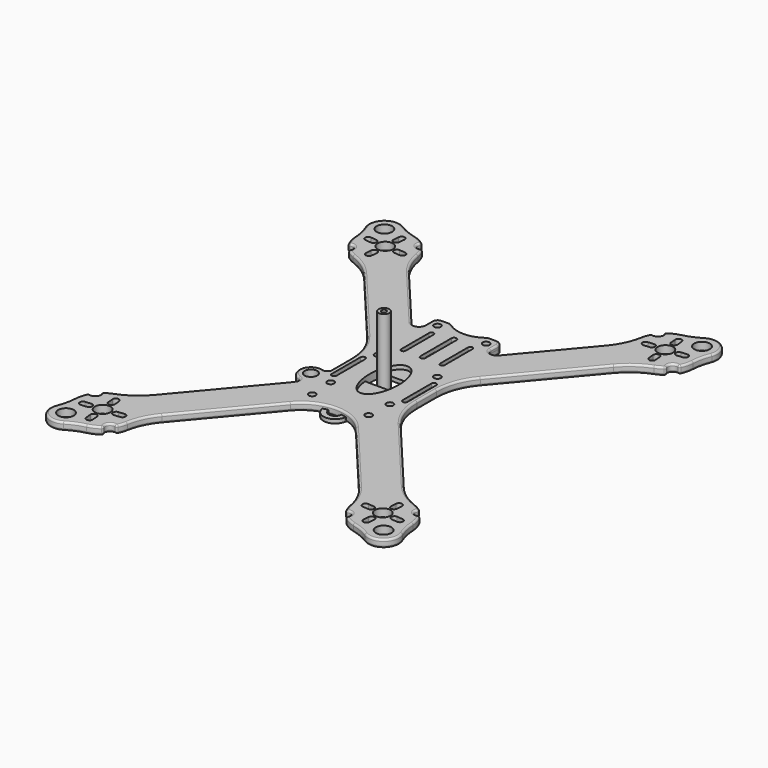
from build123d import *

# Parameters (mm, degrees)
F0_R      = 4
F0_R_2    = 1.75
F0_R_3    = 3.25
F1_DEPTH  = 4
F2_R      = 1
F4_DEPTH  = 25
F6_DEPTH  = 25
F8_DEPTH  = 25
F9_R      = 1.75
F9_R_2    = 3.25
F10_DEPTH = 2
F11_R     = 2.75
F11_R_2   = 1.25
F12_DEPTH = 35
F13_R     = 3
F15_DEPTH = 25


with BuildPart() as f1:
    # F0 (on Top) → F1 (new body)
    with BuildSketch(Plane.XY):
        with BuildLine():
            ThreePointArc((-89.0617434772, 99.3162776765), (-87.6350581485, 94.7039701662), (-86.9667023245, 89.9225360623))
            ThreePointArc((-86.9667023245, 89.9225360623), (-86.4793758867, 86.9082643751), (-85.3917451173, 84.0551292276))
            ThreePointArc((-85.3917451173, 84.0551292276), (-84.8925739132, 83.5855315092), (-84.2082817866, 83.5476079866))
            ThreePointArc((-84.2082817866, 83.5476079866), (-81.5677678239, 82.7621325082), (-81.2527459207, 80.0253375004))
            ThreePointArc((-81.2527459207, 80.0253375004), (-81.3342246225, 79.3448559582), (-80.9584413185, 78.7717234983))
            ThreePointArc((-80.9584413185, 78.7717234983), (-79.2002241246, 77.6423371812), (-77.3021125186, 76.7682585321))
            ThreePointArc((-77.3021125186, 76.7682585321), (-70.108438314, 72.9354479245), (-64.1164775039, 67.409527968))
            Line((-64.1164775039, 67.409527968), (-29.0186667064, 25.5815858579))
            ThreePointArc((-29.0186667064, 25.5815858579), (-23.8092213764, 16.5585618671), (-22, 6.2979575673))
            Line((-22, 6.2979575673), (-22, 0))
            Line((-22, 0), (-22, -6.2979575673))
            ThreePointArc((-22, -6.2979575673), (-22.0000202815, -6.3328415284), (-22.000081126, -6.3677254422))
            ThreePointArc((-22.000081126, -6.3677254422), (-22.8169100659, -7.9755627127), (-24.5957562684, -8.2723056879))
            ThreePointArc((-24.5957562684, -8.2723056879), (-32.1287124059, -12.2724390805), (-28.0506923978, -19.763516983))
            ThreePointArc((-28.0506923978, -19.763516983), (-26.7304296351, -20.9920349694), (-26.935704168, -22.7837415781))
            ThreePointArc((-26.935704168, -22.7837415781), (-27.9364881476, -24.212962377), (-29.0186667064, -25.5815858579))
            Line((-29.0186667064, -25.5815858579), (-64.1164775039, -67.409527968))
            ThreePointArc((-64.1164775039, -67.409527968), (-70.108438314, -72.9354479245), (-77.3021125186, -76.7682585321))
            ThreePointArc((-77.3021125186, -76.7682585321), (-79.2002241246, -77.6423371812), (-80.9584413185, -78.7717234983))
            ThreePointArc((-80.9584413185, -78.7717234983), (-81.3342246225, -79.3448559582), (-81.2527459207, -80.0253375004))
            ThreePointArc((-81.2527459207, -80.0253375004), (-81.5677678239, -82.7621325082), (-84.2082817866, -83.5476079866))
            ThreePointArc((-84.2082817866, -83.5476079866), (-84.8925739132, -83.5855315092), (-85.3917451173, -84.0551292276))
            ThreePointArc((-85.3917451173, -84.0551292276), (-86.4793758867, -86.9082643751), (-86.9667023245, -89.9225360623))
            ThreePointArc((-86.9667023245, -89.9225360623), (-87.6350581485, -94.7039701662), (-89.0617434772, -99.3162776765))
            ThreePointArc((-89.0617434772, -99.3162776765), (-86.7763273077, -108.4159998211), (-77.4179920365, -109.086545216))
            ThreePointArc((-77.4179920365, -109.086545216), (-73.1234971484, -106.8806156492), (-68.5307625432, -105.3921263331))
            ThreePointArc((-68.5307625432, -105.3921263331), (-65.6469077639, -104.3887806935), (-63.0259832513, -102.8222317604))
            ThreePointArc((-63.0259832513, -102.8222317604), (-62.6501999473, -102.2490993005), (-62.7316786491, -101.5686177582))
            ThreePointArc((-62.7316786491, -101.5686177582), (-62.4166567459, -98.8318227504), (-59.7761427832, -98.046347272))
            ThreePointArc((-59.7761427832, -98.046347272), (-59.0918506566, -98.0084237495), (-58.5926794524, -97.5388260311))
            ThreePointArc((-58.5926794524, -97.5388260311), (-57.7583445748, -95.5295255701), (-57.2234525085, -93.4206648569))
            ThreePointArc((-57.2234525085, -93.4206648569), (-54.8670216298, -85.9720392137), (-50.6672662494, -79.3844110213))
            Line((-50.6672662494, -79.3844110213), (-16.8529777486, -39.0861112196))
            ThreePointArc((-16.8529777486, -39.0861112196), (0, -31.2274386327), (16.8529777486, -39.0861112196))
            Line((16.8529777486, -39.0861112196), (50.6672662494, -79.3844110213))
            ThreePointArc((50.6672662494, -79.3844110213), (54.8670216298, -85.9720392137), (57.2234525085, -93.4206648569))
            ThreePointArc((57.2234525085, -93.4206648569), (57.7583445748, -95.5295255701), (58.5926794524, -97.5388260311))
            ThreePointArc((58.5926794524, -97.5388260311), (59.0918506566, -98.0084237495), (59.7761427832, -98.046347272))
            ThreePointArc((59.7761427832, -98.046347272), (62.4166567459, -98.8318227504), (62.7316786491, -101.5686177582))
            ThreePointArc((62.7316786491, -101.5686177582), (62.6501999473, -102.2490993005), (63.0259832513, -102.8222317604))
            ThreePointArc((63.0259832513, -102.8222317604), (65.6469077639, -104.3887806935), (68.5307625432, -105.3921263331))
            ThreePointArc((68.5307625432, -105.3921263331), (73.1234971484, -106.8806156492), (77.4179920365, -109.086545216))
            ThreePointArc((77.4179920365, -109.086545216), (86.7763273077, -108.4159998211), (89.0617434772, -99.3162776765))
            ThreePointArc((89.0617434772, -99.3162776765), (87.6350581485, -94.7039701662), (86.9667023245, -89.9225360623))
            ThreePointArc((86.9667023245, -89.9225360623), (86.4793758867, -86.9082643751), (85.3917451173, -84.0551292276))
            ThreePointArc((85.3917451173, -84.0551292276), (84.8925739132, -83.5855315092), (84.2082817866, -83.5476079866))
            ThreePointArc((84.2082817866, -83.5476079866), (81.5677678239, -82.7621325082), (81.2527459207, -80.0253375004))
            ThreePointArc((81.2527459207, -80.0253375004), (81.3342246225, -79.3448559582), (80.9584413185, -78.7717234983))
            ThreePointArc((80.9584413185, -78.7717234983), (79.2002241246, -77.6423371812), (77.3021125186, -76.7682585321))
            ThreePointArc((77.3021125186, -76.7682585321), (70.108438314, -72.9354479245), (64.1164775039, -67.409527968))
            Line((64.1164775039, -67.409527968), (29.0186667064, -25.5815858579))
            ThreePointArc((29.0186667064, -25.5815858579), (23.8092213764, -16.5585618671), (22, -6.2979575673))
            Line((22, -6.2979575673), (22, 0))
            Line((22, 0), (22, 6.2979575673))
            ThreePointArc((22, 6.2979575673), (23.8092213764, 16.5585618671), (29.0186667064, 25.5815858579))
            Line((29.0186667064, 25.5815858579), (64.1164775039, 67.409527968))
            ThreePointArc((64.1164775039, 67.409527968), (70.108438314, 72.9354479245), (77.3021125186, 76.7682585321))
            ThreePointArc((77.3021125186, 76.7682585321), (79.2002241246, 77.6423371812), (80.9584413185, 78.7717234983))
            ThreePointArc((80.9584413185, 78.7717234983), (81.3342246225, 79.3448559582), (81.2527459207, 80.0253375004))
            ThreePointArc((81.2527459207, 80.0253375004), (81.5677678239, 82.7621325082), (84.2082817866, 83.5476079866))
            ThreePointArc((84.2082817866, 83.5476079866), (84.8925739132, 83.5855315092), (85.3917451173, 84.0551292276))
            ThreePointArc((85.3917451173, 84.0551292276), (86.4793758867, 86.9082643751), (86.9667023245, 89.9225360623))
            ThreePointArc((86.9667023245, 89.9225360623), (87.6350581485, 94.7039701662), (89.0617434772, 99.3162776765))
            ThreePointArc((89.0617434772, 99.3162776765), (86.7763273077, 108.4159998211), (77.4179920365, 109.086545216))
            ThreePointArc((77.4179920365, 109.086545216), (73.1234971484, 106.8806156492), (68.5307625432, 105.3921263331))
            ThreePointArc((68.5307625432, 105.3921263331), (65.6469077639, 104.3887806935), (63.0259832513, 102.8222317604))
            ThreePointArc((63.0259832513, 102.8222317604), (62.6501999473, 102.2490993005), (62.7316786491, 101.5686177582))
            ThreePointArc((62.7316786491, 101.5686177582), (62.4166567459, 98.8318227504), (59.7761427832, 98.046347272))
            ThreePointArc((59.7761427832, 98.046347272), (59.0918506566, 98.0084237495), (58.5926794524, 97.5388260311))
            ThreePointArc((58.5926794524, 97.5388260311), (57.7583445748, 95.5295255701), (57.2234525085, 93.4206648569))
            ThreePointArc((57.2234525085, 93.4206648569), (54.8670216298, 85.9720392137), (50.6672662494, 79.3844110213))
            Line((50.6672662494, 79.3844110213), (22.2981333294, 45.5753949451))
            ThreePointArc((22.2981333294, 45.5753949451), (18.97393957, 44.6846799119), (17, 47.5037577742))
            Line((17, 47.5037577742), (17, 52))
            ThreePointArc((17, 52), (16.1213203436, 54.1213203436), (14, 55))
            Line((14, 55), (10.51669527, 55))
            ThreePointArc((10.51669527, 55), (9.5958514676, 54.8551789246), (8.763912725, 54.4346977944))
            ThreePointArc((8.763912725, 54.4346977944), (4.6042190121, 52.3322921432), (0, 51.6081867662))
            ThreePointArc((0, 51.6081867662), (-4.6042190121, 52.3322921432), (-8.763912725, 54.4346977944))
            ThreePointArc((-8.763912725, 54.4346977944), (-9.5958514676, 54.8551789246), (-10.51669527, 55))
            Line((-10.51669527, 55), (-14, 55))
            ThreePointArc((-14, 55), (-16.1213203436, 54.1213203436), (-17, 52))
            Line((-17, 52), (-17, 47.5037577742))
            ThreePointArc((-17, 47.5037577742), (-18.97393957, 44.6846799119), (-22.2981333294, 45.5753949451))
            Line((-22.2981333294, 45.5753949451), (-50.6672662494, 79.3844110213))
            ThreePointArc((-50.6672662494, 79.3844110213), (-54.8670216298, 85.9720392137), (-57.2234525085, 93.4206648569))
            ThreePointArc((-57.2234525085, 93.4206648569), (-57.7583445748, 95.5295255701), (-58.5926794524, 97.5388260311))
            ThreePointArc((-58.5926794524, 97.5388260311), (-59.0918506566, 98.0084237495), (-59.7761427832, 98.046347272))
            ThreePointArc((-59.7761427832, 98.046347272), (-62.4166567459, 98.8318227504), (-62.7316786491, 101.5686177582))
            ThreePointArc((-62.7316786491, 101.5686177582), (-62.6501999473, 102.2490993005), (-63.0259832513, 102.8222317604))
            ThreePointArc((-63.0259832513, 102.8222317604), (-65.6469077639, 104.3887806935), (-68.5307625432, 105.3921263331))
            ThreePointArc((-68.5307625432, 105.3921263331), (-73.1234971484, 106.8806156492), (-77.4179920365, 109.086545216))
            ThreePointArc((-77.4179920365, 109.086545216), (-86.7763273077, 108.4159998211), (-89.0617434772, 99.3162776765))
        make_face()
        with Locations((-81.6340264302, -102.2876442761)):
            Circle(F0_R, mode=Mode.SUBTRACT)
        with Locations((-71.9922122849, -90.7969776293)):
            Circle(F0_R, mode=Mode.SUBTRACT)
        with Locations((-14.5, -28)):
            Circle(F0_R_2, mode=Mode.SUBTRACT)
        with Locations((-26.3827979208, -14)):
            Circle(F0_R_3, mode=Mode.SUBTRACT)
        with Locations((-15.25, -15.25)):
            Circle(F0_R_2, mode=Mode.SUBTRACT)
        with Locations((81.6340264302, -102.2876442761)):
            Circle(F0_R, mode=Mode.SUBTRACT)
        with Locations((71.9922122849, -90.7969776293)):
            Circle(F0_R, mode=Mode.SUBTRACT)
        with Locations((14.5, -28)):
            Circle(F0_R_2, mode=Mode.SUBTRACT)
        with Locations((15.25, -15.25)):
            Circle(F0_R_2, mode=Mode.SUBTRACT)
        with BuildLine():
            Line((-19.5, 0), (-19.5, 9.25))
            ThreePointArc((-19.5, 9.25), (-19.1338834765, 10.1338834765), (-18.25, 10.5))
            ThreePointArc((-18.25, 10.5), (-17.3661165235, 10.1338834765), (-17, 9.25))
            Line((-17, 9.25), (-17, 0))
            Line((-17, 0), (-17, -9.25))
            ThreePointArc((-17, -9.25), (-17.3661165235, -10.1338834765), (-18.25, -10.5))
            ThreePointArc((-18.25, -10.5), (-19.1338834765, -10.1338834765), (-19.5, -9.25))
            Line((-19.5, -9.25), (-19.5, 0))
        make_face(mode=Mode.SUBTRACT)
        with Locations((-15.25, 15.25)):
            Circle(F0_R_2, mode=Mode.SUBTRACT)
        with Locations((-12.5, 50)):
            Circle(F0_R_2, mode=Mode.SUBTRACT)
        with Locations((-71.9922122849, 90.7969776293)):
            Circle(F0_R, mode=Mode.SUBTRACT)
        with Locations((-81.6340264302, 102.2876442761)):
            Circle(F0_R, mode=Mode.SUBTRACT)
        with BuildLine():
            Line((17, 0), (17, 9.25))
            ThreePointArc((17, 9.25), (17.3661165235, 10.1338834765), (18.25, 10.5))
            ThreePointArc((18.25, 10.5), (19.1338834765, 10.1338834765), (19.5, 9.25))
            Line((19.5, 9.25), (19.5, 0))
            Line((19.5, 0), (19.5, -9.25))
            ThreePointArc((19.5, -9.25), (19.1338834765, -10.1338834765), (18.25, -10.5))
            ThreePointArc((18.25, -10.5), (17.3661165235, -10.1338834765), (17, -9.25))
            Line((17, -9.25), (17, 0))
        make_face(mode=Mode.SUBTRACT)
        with Locations((15.25, 15.25)):
            Circle(F0_R_2, mode=Mode.SUBTRACT)
        with Locations((12.5, 50)):
            Circle(F0_R_2, mode=Mode.SUBTRACT)
        with Locations((71.9922122849, 90.7969776293)):
            Circle(F0_R, mode=Mode.SUBTRACT)
        with Locations((81.6340264302, 102.2876442761)):
            Circle(F0_R, mode=Mode.SUBTRACT)
    extrude(amount=F1_DEPTH)

    # F2
    f2_edges = [f1.edges().sort_by_distance(p)[0] for p in [
        (-54.867022, 85.972039, 4),
        (86.776327, 108.416, 0),
        (70.108438, 72.935448, 0),
        (70.108438, 72.935448, 4),
        (79.200224, 77.642337, 4),
        (81.334225, 79.344856, 4),
        (81.567768, 82.762133, 4),
        (84.892574, 83.585532, 4),
        (86.479376, 86.908264, 4),
        (87.635058, 94.70397, 4),
        (86.776327, 108.416, 4),
        (73.123497, 106.880616, 4),
        (65.646908, 104.388781, 4),
        (62.6502, 102.249099, 4),
        (62.416657, 98.831823, 4),
        (59.091851, 98.008424, 4),
        (57.758345, 95.529526, 4),
        (54.867022, 85.972039, 4),
        (36.4827, 62.479903, 4),
        (18.97394, 44.68468, 4),
        (17, 49.751879, 4),
        (16.12132, 54.12132, 4),
        (12.258348, 55, 4),
        (9.595851, 54.855179, 4),
        (0, 51.608187, 4),
        (-9.595851, 54.855179, 4),
        (-12.258348, 55, 4),
        (-16.12132, 54.12132, 4),
        (-17, 49.751879, 4),
        (-18.97394, 44.68468, 4),
        (-36.4827, 62.479903, 4),
        (-57.758345, 95.529526, 4),
        (-59.091851, 98.008424, 4),
        (-62.416657, 98.831823, 4),
        (-62.6502, 102.249099, 4),
        (-65.646908, 104.388781, 4),
        (-73.123497, 106.880616, 4),
        (-86.776327, 108.416, 4),
        (-87.635058, 94.70397, 4),
        (-86.479376, 86.908264, 4),
        (-84.892574, 83.585532, 4),
        (-81.567768, 82.762133, 4),
        (-81.334225, 79.344856, 4),
        (-79.200224, 77.642337, 4),
        (-70.108438, 72.935448, 4),
        (-46.567572, 46.495557, 4),
        (-23.809221, 16.558562, 4),
        (-22, 0, 4),
        (-22.00002, -6.332842, 4),
        (-22.81691, -7.975563, 4),
        (-32.128712, -12.272439, 4),
        (-26.73043, -20.992035, 4),
        (-27.936488, -24.212962, 4),
        (-46.567572, -46.495557, 4),
        (-70.108438, -72.935448, 4),
        (-79.200224, -77.642337, 4),
        (-81.334225, -79.344856, 4),
        (-81.567768, -82.762133, 4),
        (-84.892574, -83.585532, 4),
        (-86.479376, -86.908264, 4),
        (-87.635058, -94.70397, 4),
        (-86.776327, -108.416, 4),
        (-73.123497, -106.880616, 4),
        (-65.646908, -104.388781, 4),
        (-62.6502, -102.249099, 4),
        (-62.416657, -98.831823, 4),
        (-59.091851, -98.008424, 4),
        (-57.758345, -95.529526, 4),
        (-54.867022, -85.972039, 4),
        (-33.760122, -59.235261, 4),
        (0, -31.227439, 4),
        (33.760122, -59.235261, 4),
        (54.867022, -85.972039, 4),
        (57.758345, -95.529526, 4),
        (59.091851, -98.008424, 4),
        (62.416657, -98.831823, 4),
        (62.6502, -102.249099, 4),
        (65.646908, -104.388781, 4),
        (73.123497, -106.880616, 4),
        (86.776327, -108.416, 4),
        (87.635058, -94.70397, 4),
        (86.479376, -86.908264, 4),
        (84.892574, -83.585532, 4),
        (81.567768, -82.762133, 4),
        (81.334225, -79.344856, 4),
        (79.200224, -77.642337, 4),
        (70.108438, -72.935448, 4),
        (46.567572, -46.495557, 4),
        (23.809221, -16.558562, 4),
        (22, 0, 4),
        (23.809221, 16.558562, 4),
        (46.567572, 46.495557, 4),
        (23.809221, 16.558562, 0),
        (22, 0, 0),
        (23.809221, -16.558562, 0),
        (46.567572, -46.495557, 0),
        (70.108438, -72.935448, 0),
        (79.200224, -77.642337, 0),
        (81.334225, -79.344856, 0),
        (81.567768, -82.762133, 0),
        (84.892574, -83.585532, 0),
        (86.479376, -86.908264, 0),
        (87.635058, -94.70397, 0),
        (86.776327, -108.416, 0),
        (73.123497, -106.880616, 0),
        (65.646908, -104.388781, 0),
        (62.6502, -102.249099, 0),
        (62.416657, -98.831823, 0),
        (59.091851, -98.008424, 0),
        (57.758345, -95.529526, 0),
        (54.867022, -85.972039, 0),
        (33.760122, -59.235261, 0),
        (0, -31.227439, 0),
        (-33.760122, -59.235261, 0),
        (-54.867022, -85.972039, 0),
        (-57.758345, -95.529526, 0),
        (-59.091851, -98.008424, 0),
        (-62.416657, -98.831823, 0),
        (-62.6502, -102.249099, 0),
        (-65.646908, -104.388781, 0),
        (-73.123497, -106.880616, 0),
        (-86.776327, -108.416, 0),
        (-87.635058, -94.70397, 0),
        (-86.479376, -86.908264, 0),
        (-84.892574, -83.585532, 0),
        (-81.567768, -82.762133, 0),
        (-81.334225, -79.344856, 0),
        (-79.200224, -77.642337, 0),
        (-70.108438, -72.935448, 0),
        (-46.567572, -46.495557, 0),
        (-27.936488, -24.212962, 0),
        (-26.73043, -20.992035, 0),
        (-32.128712, -12.272439, 0),
        (-22.81691, -7.975563, 0),
        (-22.00002, -6.332842, 0),
        (-22, 0, 0),
        (-23.809221, 16.558562, 0),
        (-46.567572, 46.495557, 0),
        (-70.108438, 72.935448, 0),
        (-79.200224, 77.642337, 0),
        (-81.334225, 79.344856, 0),
        (-81.567768, 82.762133, 0),
        (-84.892574, 83.585532, 0),
        (-86.479376, 86.908264, 0),
        (-87.635058, 94.70397, 0),
        (-86.776327, 108.416, 0),
        (-73.123497, 106.880616, 0),
        (-65.646908, 104.388781, 0),
        (-62.6502, 102.249099, 0),
        (-62.416657, 98.831823, 0),
        (-59.091851, 98.008424, 0),
        (-57.758345, 95.529526, 0),
        (-54.867022, 85.972039, 0),
        (-36.4827, 62.479903, 0),
        (-18.97394, 44.68468, 0),
        (0, 51.608187, 0),
        (18.97394, 44.68468, 0),
        (36.4827, 62.479903, 0),
        (54.867022, 85.972039, 0),
        (57.758345, 95.529526, 0),
        (59.091851, 98.008424, 0),
        (62.416657, 98.831823, 0),
        (62.6502, 102.249099, 0),
        (65.646908, 104.388781, 0),
        (73.123497, 106.880616, 0),
        (87.635058, 94.70397, 0),
        (86.479376, 86.908264, 0),
        (84.892574, 83.585532, 0),
        (81.567768, 82.762133, 0),
        (81.334225, 79.344856, 0),
        (79.200224, 77.642337, 0),
        (46.567572, 46.495557, 0),
    ]]
    fillet(f2_edges, radius=F2_R)

    # F3 (on face) → F4 (cut)
    with BuildSketch(Plane(origin=(0, 0, 0), x_dir=(1, 0, 0), z_dir=(0, 0, -1))):
        with BuildLine():
            ThreePointArc((-65.3774975589, 91.8243768184), (-67.1108582642, 90.3699144899), (-65.6563959357, 88.6365537845))
            Line((-65.6563959357, 88.6365537845), (-62.6678118414, 88.3750865563))
            ThreePointArc((-62.6678118414, 88.3750865563), (-60.9344511361, 89.8295488848), (-62.3889134646, 91.5629095902))
            Line((-62.3889134646, 91.5629095902), (-65.3774975589, 91.8243768184))
        make_face()
        with BuildLine():
            Line((-72.7581442457, 100.4002764496), (-73.019611474, 97.4116923553))
            ThreePointArc((-73.019611474, 97.4116923553), (-71.5651491454, 95.67833165), (-69.8317884401, 97.1327939785))
            Line((-69.8317884401, 97.1327939785), (-69.5703212118, 100.1213780728))
            ThreePointArc((-69.5703212118, 100.1213780728), (-71.0247835404, 101.8547387781), (-72.7581442457, 100.4002764496))
        make_face()
        with BuildLine():
            Line((-81.5955111052, 90.0310456685), (-78.6069270109, 89.7695784402))
            ThreePointArc((-78.6069270109, 89.7695784402), (-76.8735663055, 91.2240407688), (-78.3280286341, 92.9574014741))
            Line((-78.3280286341, 92.9574014741), (-81.3166127284, 93.2188687024))
            ThreePointArc((-81.3166127284, 93.2188687024), (-83.0499734337, 91.7644063738), (-81.5955111052, 90.0310456685))
        make_face()
        with BuildLine():
            Line((-71.226280324, 81.1936788091), (-70.9648130958, 84.1822629033))
            ThreePointArc((-70.9648130958, 84.1822629033), (-72.4192754244, 85.9156236087), (-74.1526361297, 84.4611612801))
            Line((-74.1526361297, 84.4611612801), (-74.4141033579, 81.4725771859))
            ThreePointArc((-74.4141033579, 81.4725771859), (-72.9596410294, 79.7392164805), (-71.226280324, 81.1936788091))
        make_face()
        with BuildLine():
            Line((62.6678118414, 88.3750865563), (65.6563959357, 88.6365537845))
            ThreePointArc((65.6563959357, 88.6365537845), (67.1108582642, 90.3699144899), (65.3774975589, 91.8243768184))
            Line((65.3774975589, 91.8243768184), (62.3889134646, 91.5629095902))
            ThreePointArc((62.3889134646, 91.5629095902), (60.9344511361, 89.8295488848), (62.6678118414, 88.3750865563))
        make_face()
        with BuildLine():
            Line((70.9648130958, 84.1822629033), (71.226280324, 81.1936788091))
            ThreePointArc((71.226280324, 81.1936788091), (72.9596410294, 79.7392164805), (74.4141033579, 81.4725771859))
            Line((74.4141033579, 81.4725771859), (74.1526361297, 84.4611612801))
            ThreePointArc((74.1526361297, 84.4611612801), (72.4192754244, 85.9156236087), (70.9648130958, 84.1822629033))
        make_face()
        with BuildLine():
            Line((78.6069270109, 89.7695784402), (81.5955111052, 90.0310456685))
            ThreePointArc((81.5955111052, 90.0310456685), (83.0499734337, 91.7644063738), (81.3166127284, 93.2188687024))
            Line((81.3166127284, 93.2188687024), (78.3280286341, 92.9574014741))
            ThreePointArc((78.3280286341, 92.9574014741), (76.8735663055, 91.2240407688), (78.6069270109, 89.7695784402))
        make_face()
        with BuildLine():
            Line((69.5703212118, 100.1213780728), (69.8317884401, 97.1327939785))
            ThreePointArc((69.8317884401, 97.1327939785), (71.5651491454, 95.67833165), (73.019611474, 97.4116923553))
            Line((73.019611474, 97.4116923553), (72.7581442457, 100.4002764496))
            ThreePointArc((72.7581442457, 100.4002764496), (71.0247835404, 101.8547387781), (69.5703212118, 100.1213780728))
        make_face()
        with BuildLine():
            ThreePointArc((65.3774975589, -91.8243768184), (67.1108582642, -90.3699144899), (65.6563959357, -88.6365537845))
            Line((65.6563959357, -88.6365537845), (62.6678118414, -88.3750865563))
            ThreePointArc((62.6678118414, -88.3750865563), (60.9344511361, -89.8295488848), (62.3889134646, -91.5629095902))
            Line((62.3889134646, -91.5629095902), (65.3774975589, -91.8243768184))
        make_face()
        with BuildLine():
            Line((-62.6678118414, -88.3750865563), (-65.6563959357, -88.6365537845))
            ThreePointArc((-65.6563959357, -88.6365537845), (-67.1108582642, -90.3699144899), (-65.3774975589, -91.8243768184))
            Line((-65.3774975589, -91.8243768184), (-62.3889134646, -91.5629095902))
            ThreePointArc((-62.3889134646, -91.5629095902), (-60.9344511361, -89.8295488848), (-62.6678118414, -88.3750865563))
        make_face()
        with BuildLine():
            Line((-74.4141033579, -81.4725771859), (-74.1526361297, -84.4611612801))
            ThreePointArc((-74.1526361297, -84.4611612801), (-72.4192754244, -85.9156236087), (-70.9648130958, -84.1822629033))
            Line((-70.9648130958, -84.1822629033), (-71.226280324, -81.1936788091))
            ThreePointArc((-71.226280324, -81.1936788091), (-72.9596410294, -79.7392164805), (-74.4141033579, -81.4725771859))
        make_face()
        with BuildLine():
            Line((81.5955111052, -90.0310456685), (78.6069270109, -89.7695784402))
            ThreePointArc((78.6069270109, -89.7695784402), (76.8735663055, -91.2240407688), (78.3280286341, -92.9574014741))
            Line((78.3280286341, -92.9574014741), (81.3166127284, -93.2188687024))
            ThreePointArc((81.3166127284, -93.2188687024), (83.0499734337, -91.7644063738), (81.5955111052, -90.0310456685))
        make_face()
        with BuildLine():
            ThreePointArc((69.5703212118, -100.1213780728), (71.0247835404, -101.8547387781), (72.7581442457, -100.4002764496))
            Line((72.7581442457, -100.4002764496), (73.019611474, -97.4116923553))
            ThreePointArc((73.019611474, -97.4116923553), (71.5651491454, -95.67833165), (69.8317884401, -97.1327939785))
            Line((69.8317884401, -97.1327939785), (69.5703212118, -100.1213780728))
        make_face()
        with BuildLine():
            ThreePointArc((70.9648130958, -84.1822629033), (72.4192754244, -85.9156236087), (74.1526361297, -84.4611612801))
            Line((74.1526361297, -84.4611612801), (74.4141033579, -81.4725771859))
            ThreePointArc((74.4141033579, -81.4725771859), (72.9596410294, -79.7392164805), (71.226280324, -81.1936788091))
            Line((71.226280324, -81.1936788091), (70.9648130958, -84.1822629033))
        make_face()
        with BuildLine():
            Line((-78.6069270109, -89.7695784402), (-81.5955111052, -90.0310456685))
            ThreePointArc((-81.5955111052, -90.0310456685), (-83.0499734337, -91.7644063738), (-81.3166127284, -93.2188687024))
            Line((-81.3166127284, -93.2188687024), (-78.3280286341, -92.9574014741))
            ThreePointArc((-78.3280286341, -92.9574014741), (-76.8735663055, -91.2240407688), (-78.6069270109, -89.7695784402))
        make_face()
        with BuildLine():
            Line((-69.5703212118, -100.1213780728), (-69.8317884401, -97.1327939785))
            ThreePointArc((-69.8317884401, -97.1327939785), (-71.5651491454, -95.67833165), (-73.019611474, -97.4116923553))
            Line((-73.019611474, -97.4116923553), (-72.7581442457, -100.4002764496))
            ThreePointArc((-72.7581442457, -100.4002764496), (-71.0247835404, -101.8547387781), (-69.5703212118, -100.1213780728))
        make_face()
    extrude(amount=-F4_DEPTH, mode=Mode.SUBTRACT)

    # F5 (on face) → F6 (cut)
    with BuildSketch(Plane(origin=(0, 0, 0), x_dir=(1, 0, 0), z_dir=(0, 0, -1))):
        with BuildLine():
            ThreePointArc((1.3, -25), (0, -23.7), (-1.3, -25))
            Line((-1.3, -25), (-1.3, -45))
            ThreePointArc((-1.3, -45), (0, -46.3), (1.3, -45))
            Line((1.3, -45), (1.3, -25))
        make_face()
        with BuildLine():
            ThreePointArc((-11.15, -43), (-10, -44.15), (-8.85, -43))
            Line((-8.85, -43), (-8.85, -25))
            ThreePointArc((-8.85, -25), (-10, -23.85), (-11.15, -25))
            Line((-11.15, -25), (-11.15, -43))
        make_face()
        with BuildLine():
            Line((11.15, -43), (11.15, -25))
            ThreePointArc((11.15, -25), (10, -23.85), (8.85, -25))
            Line((8.85, -25), (8.85, -43))
            ThreePointArc((8.85, -43), (10, -44.15), (11.15, -43))
        make_face()
    extrude(amount=-F6_DEPTH, mode=Mode.SUBTRACT)

    # F7 (on face) → F8 (cut)
    with BuildSketch(Plane(origin=(0, 0, 0), x_dir=(1, 0, 0), z_dir=(0, 0, -1))):
        with BuildLine():
            add(Edge.make_bspline(
                [(0, 15), (-12.9903810568, 15), (-6.4951905284, -7.5), (0, -30), (6.4951905284, -7.5), (12.9903810568, 15), (0, 15)],
                knots=[0, 0, 0, 2.0943951024, 2.0943951024, 4.1887902048, 4.1887902048, 6.2831853072, 6.2831853072, 6.2831853072], degree=2, weights=[1, 0.5, 1, 0.5, 1, 0.5, 1]))
        make_face()
    extrude(amount=-F8_DEPTH, mode=Mode.SUBTRACT)


with BuildPart() as f10:
    # F9 (on Top) → F10 (new body)
    with BuildSketch(Plane.XY):
        with BuildLine():
            Line((-10, 55), (-14, 55))
            ThreePointArc((-14, 55), (-16.1213203436, 54.1213203436), (-17, 52))
            Line((-17, 52), (-17, 20))
            ThreePointArc((-17, 20), (-17.5857864376, 18.5857864376), (-19, 18))
            Line((-19, 18), (-19, -18))
            ThreePointArc((-19, -18), (-17.5857864376, -18.5857864376), (-17, -20))
            Line((-17, -20), (-17, -23.3095842402))
            ThreePointArc((-17, -23.3095842402), (-17.160267578, -24.0940487807), (-17.6153846154, -24.7527890894))
            ThreePointArc((-17.6153846154, -24.7527890894), (-18.0220758089, -30.800889501), (-12.0377358491, -31.7665973041))
            ThreePointArc((-12.0377358491, -31.7665973041), (-11.1241856952, -31.2007544534), (-10.1840948888, -30.6801958198))
            ThreePointArc((-10.1840948888, -30.6801958198), (-7.523159907, -30.6225109732), (-5.8635697845, -32.703295235))
            ThreePointArc((-5.8635697845, -32.703295235), (0, -37.4310730128), (5.8635697845, -32.703295235))
            ThreePointArc((5.8635697845, -32.703295235), (7.523159907, -30.6225109732), (10.1840948888, -30.6801958198))
            ThreePointArc((10.1840948888, -30.6801958198), (11.1241856952, -31.2007544534), (12.0377358491, -31.7665973041))
            ThreePointArc((12.0377358491, -31.7665973041), (18.0220758089, -30.800889501), (17.6153846154, -24.7527890894))
            ThreePointArc((17.6153846154, -24.7527890894), (17.160267578, -24.0940487807), (17, -23.3095842402))
            Line((17, -23.3095842402), (17, -20))
            ThreePointArc((17, -20), (17.5857864376, -18.5857864376), (19, -18))
            Line((19, -18), (19, 18))
            ThreePointArc((19, 18), (17.5857864376, 18.5857864376), (17, 20))
            Line((17, 20), (17, 52))
            ThreePointArc((17, 52), (16.1213203436, 54.1213203436), (14, 55))
            Line((14, 55), (10, 55))
            ThreePointArc((10, 55), (9.2928932188, 54.7071067812), (9, 54))
            Line((9, 54), (9, 37))
            ThreePointArc((9, 37), (8.1213203436, 34.8786796564), (6, 34))
            Line((6, 34), (0, 34))
            Line((0, 34), (-6, 34))
            ThreePointArc((-6, 34), (-8.1213203436, 34.8786796564), (-9, 37))
            Line((-9, 37), (-9, 54))
            ThreePointArc((-9, 54), (-9.2928932188, 54.7071067812), (-10, 55))
        make_face()
        with Locations((-14.5, -28)):
            Circle(F9_R, mode=Mode.SUBTRACT)
        with Locations((0, -31.4310730128)):
            Circle(F9_R_2, mode=Mode.SUBTRACT)
        with Locations((14.5, -28)):
            Circle(F9_R, mode=Mode.SUBTRACT)
        with Locations((-12.5, 50)):
            Circle(F9_R, mode=Mode.SUBTRACT)
        with Locations((12.5, 50)):
            Circle(F9_R, mode=Mode.SUBTRACT)
    extrude(amount=F10_DEPTH)

    # F13
    f13_edges = [f10.edges().sort_by_distance(p)[0] for p in [
        (-19, -18, 1),
        (-19, 18, 1),
        (19, 18, 1),
        (19, -18, 1),
    ]]
    fillet(f13_edges, radius=F13_R)

    # F14 (on face) → F15 (cut)
    with BuildSketch(Plane.XY.offset(2)):
        with BuildLine():
            Line((-6, 16), (6, 16))
            ThreePointArc((6, 16), (8.1213203436, 16.8786796564), (9, 19))
            Line((9, 19), (9, 25))
            ThreePointArc((9, 25), (8.1213203436, 27.1213203436), (6, 28))
            Line((6, 28), (-6, 28))
            ThreePointArc((-6, 28), (-8.1213203436, 27.1213203436), (-9, 25))
            Line((-9, 25), (-9, 19))
            ThreePointArc((-9, 19), (-8.1213203436, 16.8786796564), (-6, 16))
        make_face()
        with BuildLine():
            Line((-6, -3), (6, -3))
            ThreePointArc((6, -3), (8.1213203436, -2.1213203436), (9, 0))
            Line((9, 0), (9, 4))
            ThreePointArc((9, 4), (8.1213203436, 6.1213203436), (6, 7))
            Line((6, 7), (-6, 7))
            ThreePointArc((-6, 7), (-8.1213203436, 6.1213203436), (-9, 4))
            Line((-9, 4), (-9, 0))
            ThreePointArc((-9, 0), (-8.1213203436, -2.1213203436), (-6, -3))
        make_face()
        with BuildLine():
            ThreePointArc((4.75, -24.5), (6, -25.75), (7.25, -24.5))
            Line((7.25, -24.5), (7.25, -22))
            ThreePointArc((7.25, -22), (6, -20.75), (4.75, -22))
            Line((4.75, -22), (4.75, -24.5))
        make_face()
        with BuildLine():
            ThreePointArc((-1.25, -24.5), (0, -25.75), (1.25, -24.5))
            Line((1.25, -24.5), (1.25, -22))
            ThreePointArc((1.25, -22), (0, -20.75), (-1.25, -22))
            Line((-1.25, -22), (-1.25, -24.5))
        make_face()
        with BuildLine():
            Line((-4.75, -24.5), (-4.75, -22))
            ThreePointArc((-4.75, -22), (-6, -20.75), (-7.25, -22))
            Line((-7.25, -22), (-7.25, -24.5))
            ThreePointArc((-7.25, -24.5), (-6, -25.75), (-4.75, -24.5))
        make_face()
        with BuildLine():
            ThreePointArc((1.25, -15), (0, -13.75), (-1.25, -15))
            Line((-1.25, -15), (-1.25, -17.5))
            ThreePointArc((-1.25, -17.5), (0, -18.75), (1.25, -17.5))
            Line((1.25, -17.5), (1.25, -15))
        make_face()
        with BuildLine():
            ThreePointArc((-4.75, -15), (-6, -13.75), (-7.25, -15))
            Line((-7.25, -15), (-7.25, -17.5))
            ThreePointArc((-7.25, -17.5), (-6, -18.75), (-4.75, -17.5))
            Line((-4.75, -17.5), (-4.75, -15))
        make_face()
        with BuildLine():
            ThreePointArc((7.25, -15), (6, -13.75), (4.75, -15))
            Line((4.75, -15), (4.75, -17.5))
            ThreePointArc((4.75, -17.5), (6, -18.75), (7.25, -17.5))
            Line((7.25, -17.5), (7.25, -15))
        make_face()
        with BuildLine():
            ThreePointArc((-15.75, 3.25), (-14.5, 2), (-13.25, 3.25))
            Line((-13.25, 3.25), (-13.25, 5.75))
            ThreePointArc((-13.25, 5.75), (-14.5, 7), (-15.75, 5.75))
            Line((-15.75, 5.75), (-15.75, 3.25))
        make_face()
        with BuildLine():
            ThreePointArc((-15.75, -5.75), (-14.5, -7), (-13.25, -5.75))
            Line((-13.25, -5.75), (-13.25, -3.25))
            ThreePointArc((-13.25, -3.25), (-14.5, -2), (-15.75, -3.25))
            Line((-15.75, -3.25), (-15.75, -5.75))
        make_face()
        with BuildLine():
            ThreePointArc((-15.75, 12.25), (-14.5, 11), (-13.25, 12.25))
            Line((-13.25, 12.25), (-13.25, 14.75))
            ThreePointArc((-13.25, 14.75), (-14.5, 16), (-15.75, 14.75))
            Line((-15.75, 14.75), (-15.75, 12.25))
        make_face()
        with BuildLine():
            Line((13.25, 14.75), (13.25, 12.25))
            ThreePointArc((13.25, 12.25), (14.5, 11), (15.75, 12.25))
            Line((15.75, 12.25), (15.75, 14.75))
            ThreePointArc((15.75, 14.75), (14.5, 16), (13.25, 14.75))
        make_face()
        with BuildLine():
            Line((13.25, 5.75), (13.25, 3.25))
            ThreePointArc((13.25, 3.25), (14.5, 2), (15.75, 3.25))
            Line((15.75, 3.25), (15.75, 5.75))
            ThreePointArc((15.75, 5.75), (14.5, 7), (13.25, 5.75))
        make_face()
        with BuildLine():
            Line((13.25, -3.25), (13.25, -5.75))
            ThreePointArc((13.25, -5.75), (14.5, -7), (15.75, -5.75))
            Line((15.75, -5.75), (15.75, -3.25))
            ThreePointArc((15.75, -3.25), (14.5, -2), (13.25, -3.25))
        make_face()
    extrude(amount=-F15_DEPTH, mode=Mode.SUBTRACT)


with BuildPart() as f12:
    # F11 (on Top) → F12 (new body)
    with BuildSketch(Plane.XY):
        Circle(F11_R)
        Circle(F11_R_2, mode=Mode.SUBTRACT)
    extrude(amount=F12_DEPTH)


solid = Compound([f1.part, f10.part, f12.part])
